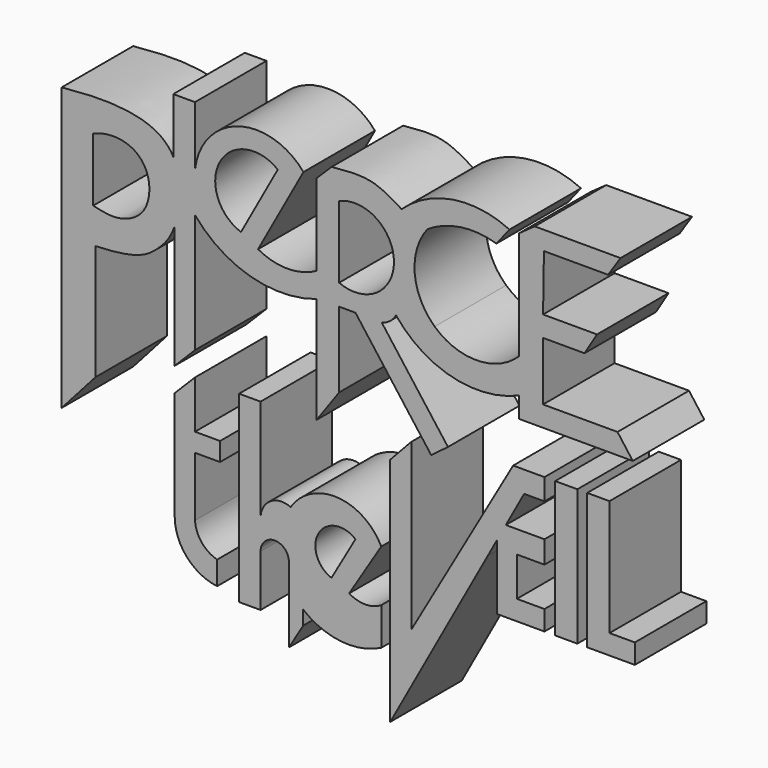
from build123d import *

# Parameters (mm, degrees)
F1_DEPTH = 12.7
F0_W     = 3.1512789428
F0_H     = 19.3154485896


# Not quite as in the source:
# - a feature names something its author has since deleted; it is built from what else it names


with BuildPart() as f1:
    # F0 (on Front) → F1 (new body)
    with BuildSketch(Plane.XZ):
        with BuildLine():
            Line((-22.7970443666, 6.0306531377), (-22.7970443666, 12.8252729774))
            Line((-22.7970443666, 12.8252729774), (-25.6827417761, 9.9253003924))
            Line((-25.6827417761, 9.9253003924), (-25.6827417761, -5.4786019027))
            ThreePointArc((-25.6827417761, -5.4786019027), (-23.9571856116, -10.0214915962), (-19.6507833898, -12.273222208))
            Line((-19.6507833898, -12.273222208), (-19.6507833898, -8.9452452958))
            ThreePointArc((-19.6507833898, -8.9452452958), (-21.848929, -7.5103998354), (-22.7970443666, -5.062604323))
            Line((-22.7970443666, -5.062604323), (-22.7970443666, 3.3960044384))
            Line((-22.7970443666, 3.3960044384), (-19.2347858101, 3.3960044384))
            Line((-19.2347858101, 3.3960044384), (-19.2347858101, 6.0306531377))
            Line((-19.2347858101, 6.0306531377), (-22.7970443666, 6.0306531377))
        make_face()
    extrude(amount=F1_DEPTH)


with BuildPart() as f1b:
    # F0 (on Front) → F1, piece 2 (new body)
    with BuildSketch(Plane.XZ):
        with Locations((29.9587789923, 6.84329262)):
            Rectangle(F0_W, F0_H)
    extrude(amount=F1_DEPTH)


with BuildPart() as f1c:
    # F0 (on Front) → F1, piece 3 (new body)
    with BuildSketch(Plane.XZ):
        Polygon((36.1009687185, 16.5010169148), (32.9344682395, 16.5010169148), (32.9344682395, -2.8144316748), (39.6982617676, -2.8144316748), (39.6982617676, 0), (36.1009687185, 0), align=None)
    extrude(amount=F1_DEPTH)


with BuildPart() as f1d:
    # F0 (on Front) → F1, piece 4 (new body)
    with BuildSketch(Plane.XZ):
        Polygon((23.2723504305, 45.8521991968), (23.2723504305, 30.4596498609), (23.2723504305, 25.5465842783), (23.2723504305, 22.6054359227), (39.4099989739, 22.6054359227), (37.2384806324, 25.5261287093), (26.6575552523, 25.5261287093), (26.6575552523, 33.8493175805), (32.5542018329, 33.8493175805), (34.3258168194, 36.7803946137), (26.6601163894, 36.7803946137), (26.783708483, 44.7525680065), (35.9011446557, 44.7525680065), (37.6653889506, 47.4146641791), (25.4651047289, 47.4146641791), align=None)
        with BuildLine():
            ThreePointArc((-22.7784111307, 38.9221281908), (-22.7881290805, 39.0132098974), (-22.7970443666, 39.1043736704))
            Line((-22.7970443666, 39.1043736704), (-22.7970443666, 38.7572443403))
            ThreePointArc((-22.7970443666, 38.7572443403), (-22.7881176358, 38.839730326), (-22.7784111307, 38.9221281908))
        make_face()
        with BuildLine():
            Line((-25.8855894208, 47.2608096898), (-25.8855894208, 39.4166894257))
            add(Edge.make_bspline(
                [(-25.8855894208, 39.4166894257), (-24.6475112984, 37.0445040507), (-24.8416415293, 33.227538681), (-25.6827417761, 30.7881627232)],
                knots=[0.4174478971, 0.4174478971, 0.4174478971, 0.4174478971, 0.6297294882, 0.6297294882, 0.6297294882, 0.6297294882], degree=3))
            Line((-25.6827417761, 30.7881627232), (-25.6827417761, 13.3388286385))
            Line((-25.6827417761, 13.3388286385), (-22.7970443666, 16.2388012235))
            Line((-22.7970443666, 16.2388012235), (-22.7970443666, 33.1357669485))
            Line((-22.7970443666, 33.1357669485), (-22.7970443666, 38.7572443403))
            Line((-22.7970443666, 38.7572443403), (-22.7970443666, 39.1043736704))
            Line((-22.7970443666, 39.1043736704), (-22.7970443666, 47.2608096898))
            Line((-22.7970443666, 47.2608096898), (-25.8855894208, 47.2608096898))
        make_face()
        with BuildLine():
            Line((-5.4981587455, 31.7787639797), (-5.4981587455, 28.2489098608))
            Line((-5.4981587455, 28.2489098608), (-5.4981587455, 13.1524559511))
            Line((-5.4981587455, 13.1524559511), (-2.3118001409, 17.6133587109))
            Line((-2.3118001409, 17.6133587109), (-2.3118001409, 28.3327493817))
            Line((-2.3118001409, 28.3327493817), (0, 28.3327493817))
            Line((0, 28.3327493817), (10.7654773061, 14.0205014217))
            Line((10.7654773061, 14.0205014217), (13.1465570685, 15.8115170761))
            Line((13.1465570685, 15.8115170761), (3.7282572594, 28.3327493817))
            add(Edge.make_bspline(
                [(3.7282572594, 28.3327493817), (4.4697086138, 28.4388605505), (5.583407823, 29.2809382081), (5.7398658246, 29.9119707197)],
                knots=[0, 0, 0, 0, 2.5574418965, 2.5574418965, 2.5574418965, 2.5574418965], degree=3))
            ThreePointArc((5.7398658246, 29.9119707197), (13.7644057738, 24.750415198), (23.2723504305, 25.5465842783))
            Line((23.2723504305, 25.5465842783), (23.2723504305, 30.4596498609))
            ThreePointArc((23.2723504305, 30.4596498609), (17.3050239314, 27.9801992486), (11.2593770027, 30.2620436996))
            ThreePointArc((11.2593770027, 30.2620436996), (8.4255284864, 35.9813750755), (10.2200610563, 42.1068221331))
            ThreePointArc((10.2200610563, 42.1068221331), (14.969664999, 43.8937045235), (20.0282521546, 43.4907376766))
            Line((20.0282521546, 43.4907376766), (21.8875091523, 45.8521991968))
            ThreePointArc((21.8875091523, 45.8521991968), (13.848280603, 46.9825580852), (6.554979831, 43.4167943895))
            add(Edge.make_bspline(
                [(-3.3745283409, 45.4758740962), (-1.4213463889, 45.669322552), (2.3339933507, 46.0412616194), (5.1862192298, 44.2678436312), (6.554979831, 43.4167943895)],
                knots=[0, 0, 0, 0, 0.520107923, 1, 1, 1, 1], degree=3))
            Line((-3.3745283409, 45.4758740962), (-5.4981587455, 43.3934754007))
            Line((-5.4981587455, 43.3934754007), (-5.4981587455, 31.7787639797))
        make_face()
        with BuildLine():
            Line((-2.3118001409, 31.334426254), (-2.3118001409, 41.5583662689))
            ThreePointArc((-2.3118001409, 41.5583662689), (5.4753586279, 36.4463962615), (-2.3118001409, 31.334426254))
        make_face(mode=Mode.SUBTRACT)
        with BuildLine():
            Line((-22.7970443666, 38.7572443403), (-22.7970443666, 33.1357669485))
            ThreePointArc((-22.7970443666, 33.1357669485), (-14.9031259742, 28.0178729436), (-5.4981587455, 28.2489098608))
            Line((-5.4981587455, 28.2489098608), (-5.4981587455, 31.7787639797))
            ThreePointArc((-5.4981587455, 31.7787639797), (-9.6662566066, 30.6964517708), (-13.8343544677, 31.7787639797))
            Line((-13.8343544677, 31.7787639797), (-7.3829540052, 43.5297638178))
            ThreePointArc((-7.3829540052, 43.5297638178), (-16.5867906437, 46.2582932174), (-22.7784111307, 38.9221281908))
            ThreePointArc((-22.7784111307, 38.9221281908), (-22.7881176358, 38.839730326), (-22.7970443666, 38.7572443403))
        make_face()
        with BuildLine():
            ThreePointArc((-16.2602435866, 33.1357669485), (-19.2483695666, 40.9652958819), (-11.0384837145, 42.6470195468))
            Line((-11.0384837145, 42.6470195468), (-16.2602435866, 33.1357669485))
        make_face(mode=Mode.SUBTRACT)
        with BuildLine():
            add(Edge.make_bspline(
                [(-41.7409986258, 42.9465435445), (-38.3140280434, 43.2744605369), (-31.9351392412, 43.6634452288), (-26.9894319336, 41.5316763702), (-25.8855894208, 39.4166894257)],
                knots=[0, 0, 0, 0, 0.2281824212, 0.4174478971, 0.4174478971, 0.4174478971, 0.4174478971], degree=3))
            Line((-41.7409986258, 42.9465435445), (-41.7409986258, 2.8491741978))
            Line((-41.7409986258, 2.8491741978), (-36.929551512, 8.2620496761))
            Line((-36.929551512, 8.2620496761), (-36.929551512, 24.6575884521))
            add(Edge.make_bspline(
                [(-25.6827417761, 30.7881627232), (-26.2896941154, 29.0278672654), (-28.5711016827, 26.5069421654), (-31.2054829086, 24.8549701927), (-36.929551512, 24.6575884521)],
                knots=[0.6297294882, 0.6297294882, 0.6297294882, 0.6297294882, 0.782915519, 1, 1, 1, 1], degree=3))
            add(Edge.make_bspline(
                [(-25.8855894208, 39.4166894257), (-24.6475112984, 37.0445040507), (-24.8416415293, 33.227538681), (-25.6827417761, 30.7881627232)],
                knots=[0.4174478971, 0.4174478971, 0.4174478971, 0.4174478971, 0.6297294882, 0.6297294882, 0.6297294882, 0.6297294882], degree=3))
        make_face()
        with BuildLine():
            Line((-37.2595600784, 29.6115428209), (-37.2595600784, 38.6322811246))
            add(Edge.make_bspline(
                [(-37.2595600784, 38.6322811246), (-35.3561267257, 39.4460260868), (-31.466902181, 39.3385766394), (-28.8684550726, 35.6553912172), (-29.5715392632, 30.735591869), (-33.7296713515, 28.7688764356), (-36.1080948778, 29.3355701334), (-37.2595600784, 29.6115428209)],
                knots=[0, 0, 0, 0, 0.2272418181, 0.4192961801, 0.62236893, 0.8172414567, 1, 1, 1, 1], degree=3))
        make_face(mode=Mode.SUBTRACT)
    extrude(amount=F1_DEPTH)


with BuildPart() as f1e:
    # F0 (on Front) → F1, piece 5 (new body)
    with BuildSketch(Plane.XZ):
        with BuildLine():
            Line((-16.5308043361, 12.8252729774), (-16.5308043361, 6.0306531377))
            Line((-16.5308043361, 6.0306531377), (-16.5308043361, -13.2438829169))
            Line((-16.5308043361, -13.2438829169), (-13.480159454, -13.2438829169))
            Line((-13.480159454, -13.2438829169), (-13.480159454, -5.8945985511))
            ThreePointArc((-13.480159454, -5.8945985511), (-11.469506193, -3.88394529), (-9.4588529319, -5.8945985511))
            Line((-9.4588529319, -5.8945985511), (-9.4588529319, -16.6180811874))
            Line((-9.4588529319, -16.6180811874), (-7.4251685292, -13.2286085109))
            Line((-7.4251685292, -13.2286085109), (-7.4251685292, -11.2130781636))
            Line((-7.4251685292, -11.2130781636), (-7.4251685292, -1.7346271779))
            ThreePointArc((-7.4251685292, -1.7346271779), (-7.9112814974, -0.0892993099), (-9.2135139302, 1.027660986))
            ThreePointArc((-9.2135139302, 1.027660986), (-12.0979918597, 0.8067553162), (-13.480159454, -1.7346271779))
            Line((-13.480159454, -1.7346271779), (-13.480159454, 12.8252729774))
            Line((-13.480159454, 12.8252729774), (-16.5308043361, 12.8252729774))
        make_face()
        with BuildLine():
            ThreePointArc((3.6680903286, 0.2758637036), (-2.5546550581, 4.3880363795), (-9.2135139302, 1.027660986))
            ThreePointArc((-9.2135139302, 1.027660986), (-7.9112814974, -0.0892993099), (-7.4251685292, -1.7346271779))
            Line((-7.4251685292, -1.7346271779), (-7.4251685292, -11.2130781636))
            ThreePointArc((-7.4251685292, -11.2130781636), (-2.0526030127, -13.4402072341), (3.6680903286, -12.3922416719))
            Line((3.6680903286, -12.3922416719), (3.6680903286, -7.0596027459))
            ThreePointArc((3.6680903286, -7.0596027459), (1.3911641285, -7.7088893182), (-0.8857620715, -7.0596027459))
            Line((-0.8857620715, -7.0596027459), (3.6680903286, 0.2758637036))
        make_face()
        with BuildLine():
            Line((0, 0), (-3.4038629383, -5.9437802993))
            ThreePointArc((-3.4038629383, -5.9437802993), (-5.2343312263, -0.9489680342), (0, 0))
        make_face(mode=Mode.SUBTRACT)
    extrude(amount=F1_DEPTH)


with BuildPart() as f1f:
    # F0 (on Front) → F1, piece 6 (new body)
    with BuildSketch(Plane.XZ):
        Polygon((26.8592257053, 16.5010169148), (22.4110993379, 16.5010169148), (7.9316468909, -8.7489113212), (7.9316468909, 14.7557211396), (4.9446239136, 11.5606354574), (4.9446239136, -21.2484076619), (18.7698199886, 3.9802147076), (20.1118197292, 6.4291351057), (20.1118197292, -2.8144316748), (26.8592257053, -2.8144316748), (26.8592257053, 0), (22.9392815381, 0), (22.9392815381, 5.5498266593), (26.8592257053, 5.5498266593), (26.8592257053, 8.7248175405), (21.3698456064, 8.7248175405), (23.9698712242, 13.4694203734), (26.8592257053, 13.4694203734), align=None)
    extrude(amount=F1_DEPTH)


solid = Compound([f1.part, f1b.part, f1c.part, f1d.part, f1e.part, f1f.part])
